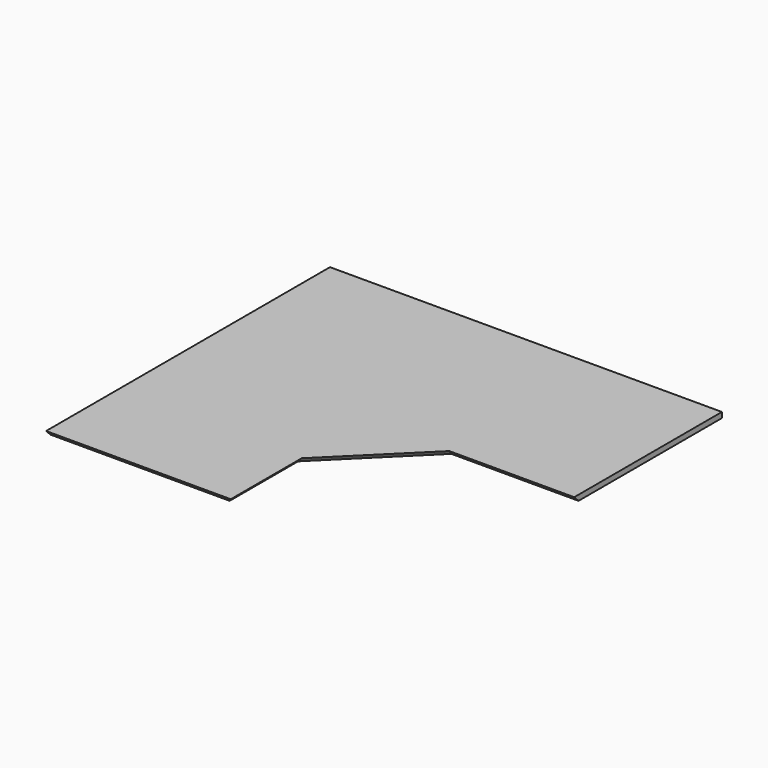
from build123d import *

# Parameters (mm, degrees)
F1_DEPTH = 19.05
F2_SIZE  = 19.04999


# Not quite as in the source:
# - a fillet or chamfer is up to 0.001 mm smaller than in the source, because OpenCascade refuses the exact size


with BuildPart() as f1:
    # F0 (on Top) → F1 (new body)
    with BuildSketch(Plane.XY):
        Polygon((0, 1244.6), (0, 0), (647.7, 0), (647.7, 311.15), (936.6773304258, 596.9), (1374.8273304258, 596.9), (1374.8273304258, 1244.6), align=None)
    extrude(amount=F1_DEPTH)

    # F2 (size 19.05 in the source; OpenCascade refuses exactly that, so slightly less here)
    f2_edges = [f1.edges().sort_by_distance(p)[0] for p in [
        (647.7, 155.575, 0),
        (792.188665, 454.025, 0),
        (1155.75233, 596.9, 0),
        (323.85, 0, 0),
    ]]
    chamfer(f2_edges, length=F2_SIZE)


solid = f1.part
